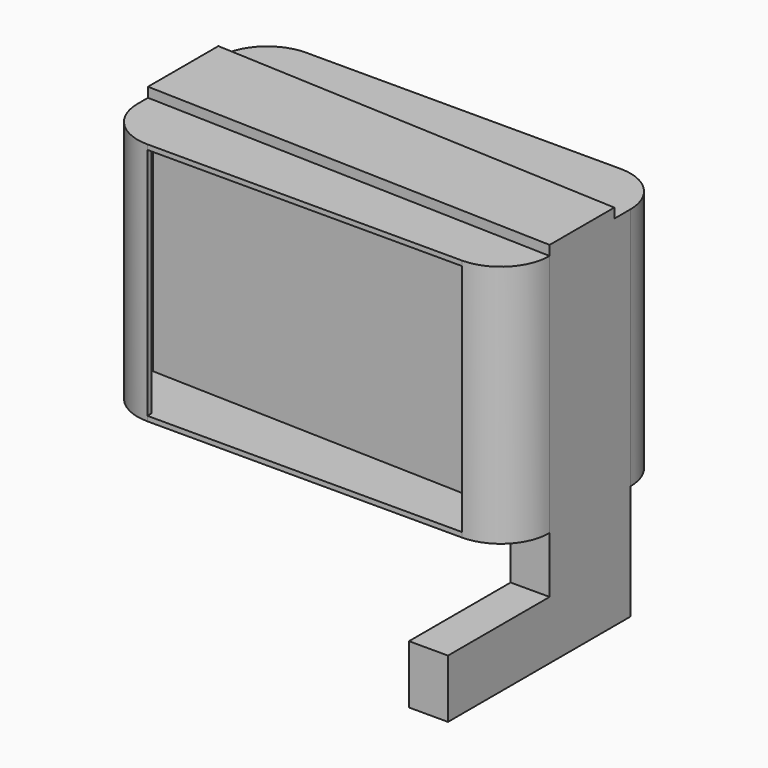
from build123d import *

# Parameters (mm, degrees)
F1_DEPTH     = 127
F2_T         = -2.54
F3_DEPTH     = 25.4
F5_DEPTH     = 132.08
F6_T         = 2.54
F6_T3_DEPTH  = 219.8768545095
F6_T5_DEPTH  = 219.7282038274
F6_T7_DEPTH  = 7.62
F6_T9_DEPTH  = 11.7497509401
F6_T11_DEPTH = 127
F6_T13_DEPTH = 214.6456904056
F6_T15_DEPTH = 5.1599103922
F6_T17_DEPTH = 7.62
F6_T19_DEPTH = 15.4153889552
F6_T21_DEPTH = 214.7908212861
F6_T23_DEPTH = 5.2038284596
F6_T26_ANGLE = 90.000000001
F6_T28_ANGLE = 90.000000001
F6_T30_ANGLE = 90.000000001
F6_T32_ANGLE = 90.000000001
F6_T34_ANGLE = 90.000000001
F6_T36_ANGLE = 90.000000001
F6_T38_ANGLE = 90.000000001
F6_T40_ANGLE = 90.000000001
F8_DEPTH     = 20.32


# Not quite as in the source:
# - a shell that OpenCascade refuses in one call is made with other operations: the cavity is built on its own and cut out


with BuildPart() as f1:
    # F0 (on Top) → F1 (new body)
    with BuildSketch(Plane.XY):
        with BuildLine():
            Line((132.6601760626, 49.2479032969), (-31.0818792045, 49.2479032969))
            ThreePointArc((-31.0818792045, 49.2479032969), (-49.0423914466, 41.8084155391), (-56.4818792045, 23.8479032969))
            Line((-56.4818792045, 23.8479032969), (158.0601760626, 23.8479032969))
            ThreePointArc((158.0601760626, 23.8479032969), (150.6206883047, 41.8084155391), (132.6601760626, 49.2479032969))
        make_face()
        Polygon((158.0601760626, 23.8479032969), (-56.4818792045, 23.8479032969), (-56.4818792045, -2.4297900897), (158.0601760626, -3.4250394454), align=None)
        Polygon((158.0601760626, -3.4250394454), (-56.4818792045, -2.4297900897), (-56.4818792045, -28.7074834764), (158.0601760626, -28.7074834764), align=None)
        with BuildLine():
            Line((158.0601760626, -28.7074834764), (-56.4818792045, -28.7074834764))
            ThreePointArc((-56.4818792045, -28.7074834764), (-49.0423914466, -46.6679957185), (-31.0818792045, -54.1074834764))
            Line((-31.0818792045, -54.1074834764), (132.6601760626, -54.1074834764))
            ThreePointArc((132.6601760626, -54.1074834764), (150.6206883047, -46.6679957185), (158.0601760626, -28.7074834764))
        make_face()
    extrude(amount=F1_DEPTH)

    # F2: a shell. OpenCascade refuses it in one call, so the cavity is built on its own and cut out:
    # the body offset inwards by the wall thickness, plus a prism from it out through each open face.
    f2_core = offset(f1.part, amount=F2_T, mode=Mode.PRIVATE)
    f2_exits = [f2_core.faces().sort_by_distance(p)[0] for p in [
        (50.789148, -51.567483, 63.5),
    ]]
    add(f2_core, mode=Mode.SUBTRACT)
    extrude(f2_exits, amount=-F2_T, mode=Mode.SUBTRACT)

    # F3 (cut): a face of the model
    f3_faces = [f1.faces().sort_by_distance(p)[0] for p in [
        (50.789148429, 46.7079032969, 63.5),
    ]]
    extrude(f3_faces, amount=-F3_DEPTH, mode=Mode.SUBTRACT)

    # F4 (on face) → F5 (join)
    with BuildSketch(Plane(origin=(0, 0, 0), x_dir=(1, 0, 0), z_dir=(0, 0, -1))):
        Polygon((158.0601760626, 28.7074834764), (-56.4818792045, 21.957822144), (-56.4818792045, -23.8479032969), (158.0601760626, -13.3886858821), align=None)
    extrude(amount=-F5_DEPTH)

    # F6: shell of thickness 2.54, made by hand


with BuildPart() as f6_core1:
    # F6_t2: copy of F1
    add(f1.part)

    # the walls: a layer under each face that stays
    f6_faces = [f6_core1.faces().sort_by_distance(p)[0] for p in [
        (-49.0423914466, 41.8084155391, 63.5),
        (50.789148429, 31.3182945895, 127),
        (50.789148429, 18.6182945895, 129.54),
        (50.789148429, -2.4297900897, 132.08),
        (50.789148429, -25.3326528102, 129.54),
        (50.789148429, -38.0326528102, 127),
        (-49.0423914466, -46.6679957185, 63.5),
        (-31.0818792045, -52.8374834764, 63.5),
        (-47.2463402224, -44.8719444943, 63.5),
        (-53.9418792045, -25.3726080063, 63.5),
        (50.789148429, -25.3326528102, 63.5),
        (155.5201760626, -28.6675282803, 63.5),
        (148.8246370805, -44.8719444943, 63.5),
        (132.6601760626, -52.8374834764, 63.5),
        (50.789148429, -38.0726080063, 124.46),
        (50.789148429, -38.0726080063, 2.54),
        (50.789148429, -54.1074834764, 1.27),
        (50.789148429, -54.1074834764, 125.73),
        (150.6206883047, -46.6679957185, 63.5),
        (158.0601760626, -2.4297900897, 66.04),
        (150.6206883047, 41.8084155391, 63.5),
        (132.6601760626, 47.9779032969, 63.5),
        (50.789148429, 31.3802088193, 2.54),
        (-47.2463402224, 40.0123643149, 63.5),
        (-53.9418792045, 23.7859890671, 63.5),
        (50.789148429, 18.6182945895, 63.5),
        (155.5201760626, 18.6802088193, 63.5),
        (50.789148429, 31.3802088193, 124.46),
        (148.8246370805, 40.0123643149, 63.5),
        (-56.4818792045, -2.4297900897, 66.04),
        (50.789148429, 49.2479032969, 125.73),
        (-31.0818792045, 47.9779032969, 63.5),
        (50.789148429, 49.2479032969, 1.27),
    ]]
    thicken(f6_faces, amount=-F6_T, mode=Mode.SUBTRACT)

    # F6_s4 → F6_t3 (cut)
    with BuildSketch(Plane(origin=(159.571223823, -7.779314508, 0), x_dir=(0, 0, 1), z_dir=(-0.9988137664, 0.0486935316, 0))):
        Polygon((127.0254, 21.0947119453), (124.46, 21.0693119453), (124.46, 18.5293119453), (127, 18.5293119453), align=None)
    extrude(amount=F6_T3_DEPTH, mode=Mode.SUBTRACT)

    # F6_s6 → F6_t5 (cut)
    with BuildSketch(Plane(origin=(-58.2746464734, 1.8333660851, 0), x_dir=(0, 0, 1), z_dir=(0.9995054766, -0.0314452262, 0))):
        Polygon((127.0254, 23.7484489574), (127, 21.1830489574), (124.46, 21.1830489574), (124.46, 23.7230489574), align=None)
    extrude(amount=F6_T5_DEPTH, mode=Mode.SUBTRACT)

    # F6_s8 → F6_t7 (cut)
    with BuildSketch(Plane.XZ.offset(49.0274834764)):
        Polygon((-31.0564792045, 2.5654), (-33.6218792045, 2.54), (-33.6218792045, 0), (-31.0818792045, 0), align=None)
        Polygon((-31.0564792045, 124.4346), (-33.6218792045, 124.46), (-33.6218792045, 127), (-31.0818792045, 127), align=None)
        Polygon((132.6347760626, 2.5654), (135.2001760626, 2.54), (135.2001760626, 0), (132.6601760626, 0), align=None)
        Polygon((132.6347760626, 124.4346), (135.2001760626, 124.46), (135.2001760626, 127), (132.6601760626, 127), align=None)
    extrude(amount=F6_T7_DEPTH, mode=Mode.SUBTRACT)

    # F6_s10 → F6_t9 (cut)
    with BuildSketch(Plane.XZ.offset(19.4977325363)):
        Polygon((-53.9164792045, 2.5654), (-56.4818792045, 2.54), (-56.4818792045, 0), (-53.9418792045, 0), align=None)
        Polygon((-53.9164792045, 124.4346), (-56.4818792045, 124.46), (-56.4818792045, 127), (-53.9418792045, 127), align=None)
    extrude(amount=F6_T9_DEPTH, mode=Mode.SUBTRACT)

    # F6_s12 → F6_t11 (cut)
    with BuildSketch(Plane.XY):
        Polygon((-53.9172779133, -22.0631199754), (-56.4818792045, -22.0377325363), (-56.4818792045, -19.4165654331), (-53.8620083299, -19.4989886257), align=None)
        Polygon((155.4939773538, -28.6529605233), (155.6000469372, -26.0888291736), (158.0601760626, -26.1662267655), (158.0601760626, -28.6275730842), align=None)
        Polygon((-53.9152423888, 23.749444707), (-56.4818792045, 23.7240748373), (-56.4818792045, 21.3048866852), (-54.0655607747, 21.1870878706), align=None)
        Polygon((155.4960128783, 13.5378842114), (155.3964944924, 10.975527375), (158.0601760626, 10.8456692704), (158.0601760626, 13.5125143417), align=None)
    extrude(amount=F6_T11_DEPTH, mode=Mode.SUBTRACT)

    # F6_s14 → F6_t13 (cut)
    with BuildSketch(Plane(origin=(-55.7346464734, 1.7534556929, 0), x_dir=(0, 0, 1), z_dir=(0.9995054766, -0.0314452262, 0))):
        Polygon((124.4346, 23.7484489574), (124.46, 21.1830489574), (127, 21.1830489574), (127, 23.7230489574), align=None)
        Polygon((2.5654, 23.7484489574), (2.54, 21.1830489574), (0, 21.1830489574), (0, 23.7230489574), align=None)
    extrude(amount=F6_T13_DEPTH, mode=Mode.SUBTRACT)

    # F6_s16 → F6_t15 (cut)
    with BuildSketch(Plane.XZ.offset(26.0875730842)):
        Polygon((155.4947760626, 124.4346), (158.0601760626, 124.46), (158.0601760626, 127), (155.5201760626, 127), align=None)
        Polygon((155.4947760626, 2.5654), (158.0601760626, 2.54), (158.0601760626, 0), (155.5201760626, 0), align=None)
    extrude(amount=F6_T15_DEPTH, mode=Mode.SUBTRACT)

    # F6_s18 → F6_t17 (cut)
    with BuildSketch(Plane.XZ.offset(-51.7879032969)):
        Polygon((132.6347760626, 124.4346), (135.2001760626, 124.46), (135.2001760626, 127), (132.6601760626, 127), align=None)
        Polygon((132.6347760626, 2.5654), (135.2001760626, 2.54), (135.2001760626, 0), (132.6601760626, 0), align=None)
        Polygon((-31.0564792045, 2.5654), (-31.0818792045, 0), (-33.6218792045, 0), (-33.6218792045, 2.54), align=None)
        Polygon((-31.0564792045, 124.4346), (-31.0818792045, 127), (-33.6218792045, 127), (-33.6218792045, 124.46), align=None)
    extrude(amount=F6_T17_DEPTH, mode=Mode.SUBTRACT)

    # F6_s20 → F6_t19 (cut)
    with BuildSketch(Plane.XZ.offset(-26.3879032969)):
        Polygon((155.4947760626, 2.5654), (155.5201760626, 0), (158.0601760626, 0), (158.0601760626, 2.54), align=None)
        Polygon((155.4947760626, 124.4346), (158.0601760626, 124.46), (158.0601760626, 127), (155.5201760626, 127), align=None)
    extrude(amount=F6_T19_DEPTH, mode=Mode.SUBTRACT)

    # F6_s22 → F6_t21 (cut)
    with BuildSketch(Plane(origin=(157.031223823, -7.6554860484, 0), x_dir=(0, 0, 1), z_dir=(-0.9988137664, 0.0486935316, 0))):
        Polygon((2.5654, 21.0947119453), (0, 21.0693119453), (0, 18.5293119453), (2.54, 18.5293119453), align=None)
        Polygon((124.4346, 21.0947119453), (124.46, 18.5293119453), (127, 18.5293119453), (127, 21.0693119453), align=None)
    extrude(amount=F6_T21_DEPTH, mode=Mode.SUBTRACT)

    # F6_s24 → F6_t23 (cut)
    with BuildSketch(Plane.XZ.offset(-26.3879032969)):
        Polygon((-53.9164792045, 2.5654), (-53.9418792045, 0), (-56.4818792045, 0), (-56.4818792045, 2.54), align=None)
        Polygon((-53.9164792045, 124.4346), (-56.4818792045, 124.46), (-56.4818792045, 127), (-53.9418792045, 127), align=None)
    extrude(amount=F6_T23_DEPTH, mode=Mode.SUBTRACT)

    # F6_s25 → F6_t26 (revolve, cut)
    with BuildSketch(Plane.YZ.offset(-31.0818792045)):
        Polygon((-51.5420834764, 124.4346), (-54.1074834764, 124.46), (-54.1074834764, 127), (-51.5674834764, 127), align=None)
    revolve(axis=Axis((-31.0818792045, -28.7074834764, 124.46), (0, 0, -1)), revolution_arc=F6_T26_ANGLE, mode=Mode.SUBTRACT)

    # F6_s27 → F6_t28 (revolve, cut)
    with BuildSketch(Plane.YZ.offset(-31.0818792045)):
        Polygon((-51.5420834764, 2.5654), (-54.1074834764, 2.54), (-54.1074834764, 0), (-51.5674834764, 0), align=None)
    revolve(axis=Axis((-31.0818792045, -28.7074834764, 2.54), (0, 0, -1)), revolution_arc=F6_T28_ANGLE, mode=Mode.SUBTRACT)

    # F6_s29 → F6_t30 (revolve, cut)
    with BuildSketch(Plane.XZ.offset(28.7074834764)):
        Polygon((155.4947760626, 124.4346), (158.0601760626, 124.46), (158.0601760626, 127), (155.5201760626, 127), align=None)
    revolve(axis=Axis((132.6601760626, -28.7074834764, 124.46), (0, 0, -1)), revolution_arc=F6_T30_ANGLE, mode=Mode.SUBTRACT)

    # F6_s31 → F6_t32 (revolve, cut)
    with BuildSketch(Plane.XZ.offset(28.7074834764)):
        Polygon((155.4947760626, 2.5654), (158.0601760626, 2.54), (158.0601760626, 0), (155.5201760626, 0), align=None)
    revolve(axis=Axis((132.6601760626, -28.7074834764, 2.54), (0, 0, -1)), revolution_arc=F6_T32_ANGLE, mode=Mode.SUBTRACT)

    # F6_s33 → F6_t34 (revolve, cut)
    with BuildSketch(Plane.YZ.offset(132.6601760626)):
        Polygon((46.6825032969, 2.5654), (46.7079032969, 0), (49.2479032969, 0), (49.2479032969, 2.54), align=None)
    revolve(axis=Axis((132.6601760626, 23.8479032969, 2.54), (0, 0, -1)), revolution_arc=F6_T34_ANGLE, mode=Mode.SUBTRACT)

    # F6_s35 → F6_t36 (revolve, cut)
    with BuildSketch(Plane.XZ.offset(-23.8479032969)):
        Polygon((-53.9164792045, 2.5654), (-53.9418792045, 0), (-56.4818792045, 0), (-56.4818792045, 2.54), align=None)
    revolve(axis=Axis((-31.0818792045, 23.8479032969, 2.54), (0, 0, -1)), revolution_arc=F6_T36_ANGLE, mode=Mode.SUBTRACT)

    # F6_s37 → F6_t38 (revolve, cut)
    with BuildSketch(Plane.XZ.offset(-23.8479032969)):
        Polygon((-53.9164792045, 124.4346), (-56.4818792045, 124.46), (-56.4818792045, 127), (-53.9418792045, 127), align=None)
    revolve(axis=Axis((-31.0818792045, 23.8479032969, 124.46), (0, 0, -1)), revolution_arc=F6_T38_ANGLE, mode=Mode.SUBTRACT)

    # F6_s39 → F6_t40 (revolve, cut)
    with BuildSketch(Plane.YZ.offset(132.6601760626)):
        Polygon((46.6825032969, 124.4346), (46.7079032969, 127), (49.2479032969, 127), (49.2479032969, 124.46), align=None)
    revolve(axis=Axis((132.6601760626, 23.8479032969, 124.46), (0, 0, -1)), revolution_arc=F6_T40_ANGLE, mode=Mode.SUBTRACT)


with BuildPart() as f1_1:
    add(f1.part)

    # what is left inside the walls is the cavity
    f6_cavity = [f6_core1.part.solids().sort_by_distance(p)[0] for p in [
        (15.877569, 17.751835, 64.77),
    ]]
    add(f6_cavity, mode=Mode.SUBTRACT)

    # F7 (on face) → F8 (join)
    with BuildSketch(Plane.YZ.offset(158.0601760626)):
        Polygon((23.8479032969, -59.71023524), (23.8479032969, 0), (-28.7074834764, 0), (-28.7074834764, -29.3008414079), (-94.8645432204, -29.3008414079), (-94.8645432204, -59.71023524), align=None)
    extrude(amount=-F8_DEPTH)


solid = f1_1.part
